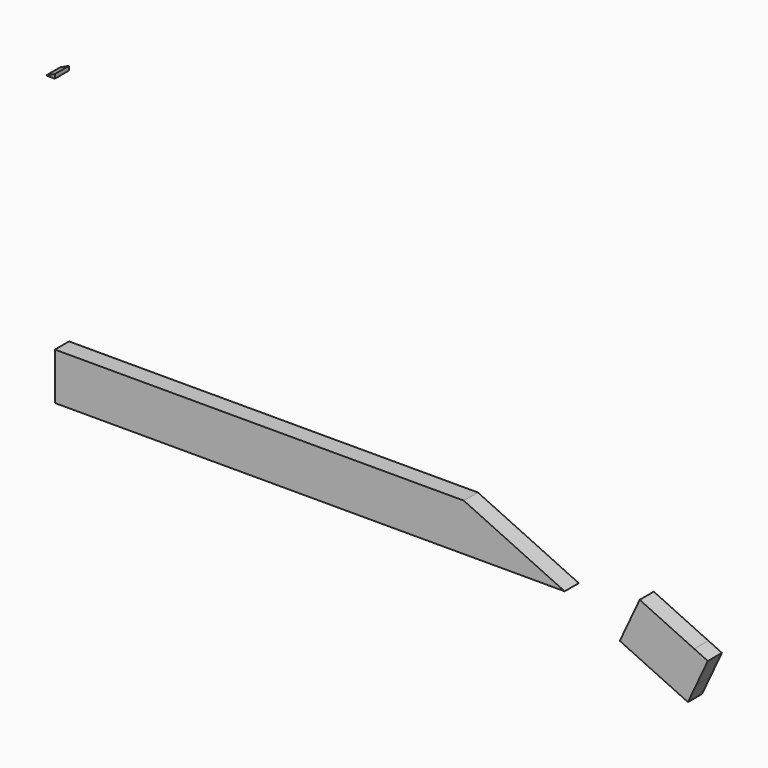
from build123d import *

# Parameters (mm, degrees)
F1_DEPTH = 45


# Not quite as in the source:
# - a feature names something its author has since deleted; it is built from what else it names


with BuildPart() as f1:
    # F0 (on Front) → F1 (new body)
    with BuildSketch(Plane.XZ):
        Polygon((1440.5510948329, 81.0138275128), (1614.2858085911, 0), (1635.4167216782, 45.3153893518), (1665, 108.7569344444), (1630.5603040926, 124.8164283905), (1491.2652862418, 189.7707619572), align=None)
    extrude(amount=F1_DEPTH)


with BuildPart() as f1b:
    # F0 (on Front) → F1, piece 2 (new body)
    with BuildSketch(Plane.XZ):
        Polygon((1210, 146.5538793955), (1300, 146.5538793955), (1042.6591695389, 266.5538793955), (0, 266.5538793955), (0, 146.5538793955), align=None)
    extrude(amount=F1_DEPTH)


with BuildPart() as f1c:
    # F0 (on Front) → F1, piece 3 (new body)
    with BuildSketch(Plane.XZ):
        Polygon((-22.5, 874.667262964), (0, 874.667262964), (0, 885.1591852725), align=None)
    extrude(amount=F1_DEPTH)


solid = Compound([f1.part, f1b.part, f1c.part])
